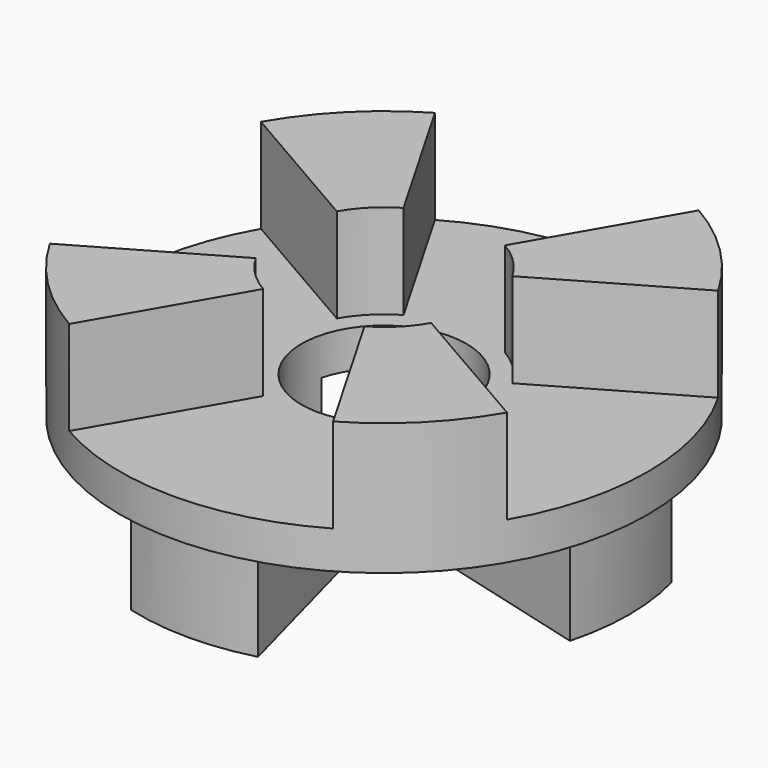
from build123d import *

# Parameters (mm, degrees)
F3_DEPTH = 127
F5_DEPTH = 127


with BuildPart() as f1:
    # F0 (on Front) → F1 (revolve)
    with BuildSketch(Plane.XZ):
        Polygon((136.525, 177.8), (111.125, 177.8), (111.125, 0), (330.2, 0), (330.2, 127), (355.6, 127), (355.6, 304.8), (136.525, 304.8), align=None)
    revolve(axis=Axis((0, 0, 359.9156904304), (0, 0, 1)))

    # F2 (on face) → F3 (cut)
    with BuildSketch(Plane.XY.offset(304.8)):
        with BuildLine():
            ThreePointArc((-307.9586335857, 177.8), (-355.6, 0), (-307.9586335857, -177.8))
            Line((-307.9586335857, -177.8), (-118.2341182517, -68.2625))
            ThreePointArc((-118.2341182517, -68.2625), (-136.525, 0), (-118.2341182517, 68.2625))
            Line((-118.2341182517, 68.2625), (-307.9586335857, 177.8))
        make_face()
        with BuildLine():
            Line((-68.2625, -118.2341182517), (-177.8, -307.9586335857))
            ThreePointArc((-177.8, -307.9586335857), (0, -355.6), (177.8, -307.9586335857))
            Line((177.8, -307.9586335857), (68.2625, -118.2341182517))
            ThreePointArc((68.2625, -118.2341182517), (0, -136.525), (-68.2625, -118.2341182517))
        make_face()
        with BuildLine():
            ThreePointArc((177.8, 307.9586335857), (0, 355.6), (-177.8, 307.9586335857))
            Line((-177.8, 307.9586335857), (-68.2625, 118.2341182517))
            ThreePointArc((-68.2625, 118.2341182517), (0, 136.525), (68.2625, 118.2341182517))
            Line((68.2625, 118.2341182517), (177.8, 307.9586335857))
        make_face()
        with BuildLine():
            Line((307.9586335857, 177.8), (118.2341182517, 68.2625))
            ThreePointArc((118.2341182517, 68.2625), (131.8730234341, 35.3352701326), (136.525, 0))
            ThreePointArc((136.525, 0), (131.8730234341, -35.3352701326), (118.2341182517, -68.2625))
            Line((118.2341182517, -68.2625), (307.9586335857, -177.8))
            ThreePointArc((307.9586335857, -177.8), (343.4832238284, -92.0360524385), (355.6, 0))
            ThreePointArc((355.6, 0), (343.4832238284, 92.0360524385), (307.9586335857, 177.8))
        make_face()
        with BuildLine():
            ThreePointArc((355.6, 0), (343.4832238284, -92.0360524385), (307.9586335857, -177.8))
            Line((307.9586335857, -177.8), (329.9556788419, -190.5))
            ThreePointArc((329.9556788419, -190.5), (381, 0), (329.9556788419, 190.5))
            Line((329.9556788419, 190.5), (307.9586335857, 177.8))
            ThreePointArc((307.9586335857, 177.8), (343.4832238284, 92.0360524385), (355.6, 0))
        make_face()
    extrude(amount=-F3_DEPTH, mode=Mode.SUBTRACT)

    # F4 (on face) → F5 (cut)
    with BuildSketch(Plane(origin=(0, 0, 0), x_dir=(1, 0, 0), z_dir=(0, 0, -1))):
        with BuildLine():
            Line((-28.761266387, 107.3385074464), (-85.4620486929, 318.9487078407))
            ThreePointArc((-85.4620486928, 318.9487078407), (-233.4866591478, 233.4866591478), (-318.9487078407, 85.4620486929))
            Line((-318.9487078407, 85.4620486929), (-107.3385074464, 28.761266387))
            ThreePointArc((-107.3385074464, 28.761266387), (-78.5772410594, 78.5772410594), (-28.761266387, 107.3385074464))
        make_face()
        with BuildLine():
            Line((107.3385074464, 28.761266387), (318.9487078407, 85.4620486929))
            ThreePointArc((318.9487078406, 85.4620486929), (233.4866591478, 233.4866591478), (85.4620486928, 318.9487078407))
            Line((85.4620486929, 318.9487078407), (28.761266387, 107.3385074464))
            ThreePointArc((28.761266387, 107.3385074464), (78.5772410594, 78.5772410594), (107.3385074464, 28.761266387))
        make_face()
        with BuildLine():
            ThreePointArc((85.4620486928, -318.9487078407), (233.4866591478, -233.4866591478), (318.9487078406, -85.4620486929))
            Line((318.9487078407, -85.4620486929), (107.3385074464, -28.761266387))
            ThreePointArc((107.3385074464, -28.761266387), (78.5772410594, -78.5772410594), (28.761266387, -107.3385074464))
            Line((28.761266387, -107.3385074464), (85.4620486929, -318.9487078407))
        make_face()
        with BuildLine():
            ThreePointArc((-318.9487078407, -85.4620486929), (-233.4866591478, -233.4866591478), (-85.4620486928, -318.9487078407))
            Line((-85.4620486929, -318.9487078407), (-28.761266387, -107.3385074464))
            ThreePointArc((-28.761266387, -107.3385074464), (-78.5772410594, -78.5772410594), (-107.3385074464, -28.761266387))
            Line((-107.3385074464, -28.761266387), (-318.9487078407, -85.4620486929))
        make_face()
    extrude(amount=-F5_DEPTH, mode=Mode.SUBTRACT)


solid = f1.part
